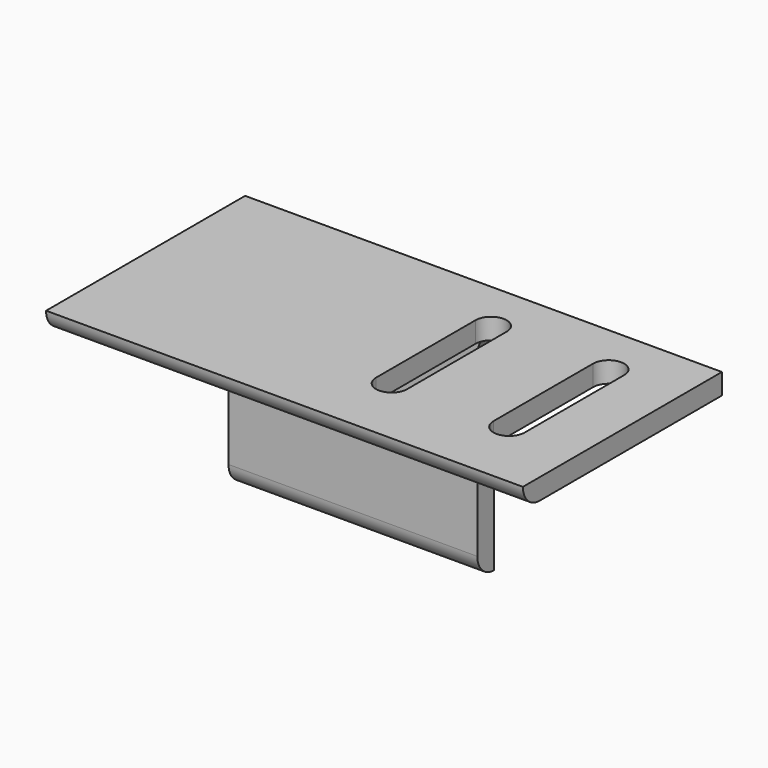
from build123d import *

# Parameters (mm, degrees)
F0_W     = 73.025
F0_H     = 38.1
F1_DEPTH = 3.175
F2_W     = 73.025
F2_H     = 34.925
F3_DEPTH = 3.175
F5_D     = 3.2
F5_DEPTH = 34.925
F5_TIP   = 0.9613769904
F7_DEPTH = 3.176
F8_W     = 34.925
F8_H     = 34.925
F9_DEPTH = 3.176
F10_R    = 3.17499
F11_R    = 4.7625


# Not quite as in the source:
# - a fillet or chamfer is up to 0.001 mm smaller than in the source, because OpenCascade refuses the exact size


with BuildPart() as f1:
    # F0 (on Front) → F1 (new body)
    with BuildSketch(Plane.XZ):
        Rectangle(F0_W, F0_H)
    extrude(amount=F1_DEPTH)

    # F2 (on face) → F3 (join)
    with BuildSketch(Plane.XY.offset(19.05)):
        with Locations((0, -20.6375)):
            Rectangle(F2_W, F2_H)
    extrude(amount=-F3_DEPTH)

    # F5
    with Locations(Plane.XZ.offset(3.175)):
        with Locations((-27.78125, -4.05)):
            Hole(F5_D / 2, depth=F5_DEPTH)
            with Locations((0, 0, -(F5_DEPTH + F5_TIP / 2))):  # 118° drill point
                Cone(0, F5_D / 2, F5_TIP, mode=Mode.SUBTRACT)

    # F6 (on face) → F7 (cut, through all)
    with BuildSketch(Plane(origin=(0, 0, 15.875), x_dir=(1, 0, 0), z_dir=(0, 0, -1))):
        with BuildLine():
            ThreePointArc((5.13125, 7.9375), (7.5125, 5.55625), (9.89375, 7.9375))
            Line((9.89375, 7.9375), (9.89375, 26.9875))
            ThreePointArc((9.89375, 26.9875), (7.5125, 29.36875), (5.13125, 26.9875))
            Line((5.13125, 26.9875), (5.13125, 7.9375))
        make_face()
        with BuildLine():
            ThreePointArc((23.13125, 7.9375), (25.5125, 5.55625), (27.89375, 7.9375))
            Line((27.89375, 7.9375), (27.89375, 26.9875))
            ThreePointArc((27.89375, 26.9875), (25.5125, 29.36875), (23.13125, 26.9875))
            Line((23.13125, 26.9875), (23.13125, 7.9375))
        make_face()
    extrude(amount=-F7_DEPTH, mode=Mode.SUBTRACT)

    # F8 (on face) → F9 (cut, through all)
    with BuildSketch(Plane.XZ.offset(3.175)):
        with Locations((19.05, -1.5875)):
            Rectangle(F8_W, F8_H)
    extrude(amount=-F9_DEPTH, mode=Mode.SUBTRACT)

    # F10 (radius 3.175 in the source; OpenCascade refuses exactly that, so slightly less here)
    f10_edges = [f1.edges().sort_by_distance(p)[0] for p in [
        (0, -38.1, 15.875),
        (-17.4625, -3.175, -19.05),
    ]]
    fillet(f10_edges, radius=F10_R)

    # F11
    f11_edges = [f1.edges().sort_by_distance(p)[0] for p in [
        (1.5875, -1.5875, 15.875),
    ]]
    fillet(f11_edges, radius=F11_R)


solid = f1.part
